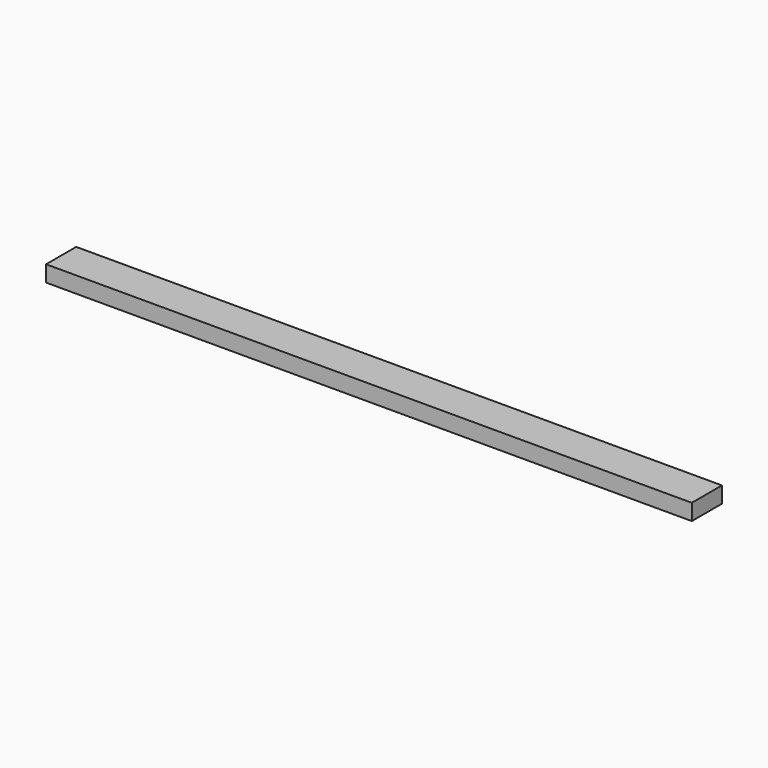
from build123d import *

# Parameters (mm, degrees)
F1_W     = 88.9
F1_H     = 38.1
F2_DEPTH = 762


# Not quite as in the source:
# - a variable given as a bare number and used for a length is read in inches; the dataset says mm whatever the document's units were


with BuildPart() as f2:
    # F1 (on Right) → F2 (new body, symmetric)
    with BuildSketch(Plane.YZ):
        Rectangle(F1_W, F1_H)
    extrude(amount=F2_DEPTH, both=True)


solid = f2.part
